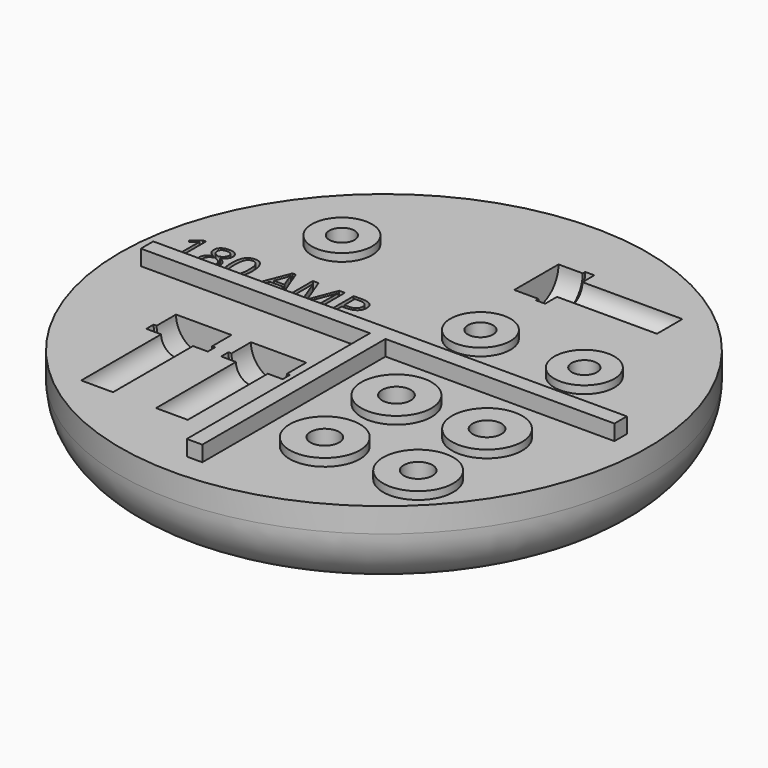
from build123d import *

# Parameters (mm, degrees)
F0_W         = 43
F0_H         = 2
F2_R         = 43.5
F3_DEPTH     = 2
F4_W         = 4
F4_H         = 3.0127849464
F4_H_2       = 58.9872150536
F5_DEPTH     = 4
F6_TEXT_SIZE = 11.6792921391
F7_DEPTH     = 2
F9_R         = 7.75
F10_DEPTH    = 2
F8_R         = 7.75
F11_DEPTH    = 2
F12_R        = 3.25
F13_DEPTH    = 19
F14_R        = 7.75
F15_DEPTH    = 2
F16_R        = 3.25
F17_DEPTH    = 19
F18_R        = 7.75
F19_DEPTH    = 2
F20_R        = 3.25
F21_DEPTH    = 19
F28_R        = 9.05
F32_DEPTH    = 2
F29_R        = 9.05
F30_R        = 9.05
F33_DEPTH    = 2
F31_R        = 9.05
F34_DEPTH    = 2
F35_R        = 3.7
F38_R        = 3.7
F37_R        = 3.7
F36_R        = 3.7
F39_DEPTH    = 19


# Not quite as in the source:
# - Text() gives the source's letters only with a copy of the font that has no kerning and outlines rounded to 1/6400 em; it was checked with that copy


with BuildPart() as f1:
    # F0 (on Front) → F1 (revolve)
    with BuildSketch(Plane.XZ):
        with BuildLine():
            Line((0, -19.3), (0, 0))
            Line((0, 0), (-68, 0))
            Line((-68, 0), (-68, -6.3))
            ThreePointArc((-68, -6.3), (-63.6066017178, -16.9066017178), (-53, -21.3))
            Line((-53, -21.3), (-43, -21.3))
            Line((-43, -21.3), (-43, -19.3))
            Line((-43, -19.3), (0, -19.3))
        make_face()
        with Locations((-21.5, -20.3)):
            Rectangle(F0_W, F0_H)
    revolve(axis=Axis((0, 0, -20.3), (0, 0, 1)))

    # F2 (on face) → F3 (cut)
    with BuildSketch(Plane(origin=(0, 0, -21.3), x_dir=(1, 0, 0), z_dir=(0, 0, -1))):
        Circle(F2_R)
    extrude(amount=-F3_DEPTH, mode=Mode.SUBTRACT)

    # F4 (on face) → F5 (join)
    with BuildSketch(Plane.XY):
        Polygon((-2, -2), (-2, 1.0127849464), (2, 1.0127849464), (2, -2), (60.9872150536, -2), (60.9872150536, 2), (-61.02, 2), (-61.02, -2), align=None)
        with Locations((0, -0.4936075268)):
            Rectangle(F4_W, F4_H)
        with Locations((0, -31.4936075268)):
            Rectangle(F4_W, F4_H_2)
    extrude(amount=F5_DEPTH)

    # F6 (on face) → F7 (cut)
    with BuildSketch(Plane.XY):
        with Locations((-61.5909136832, 6.2500005588)):
            Text('180 AMP', F6_TEXT_SIZE, font='Open Sans', text_align=(TextAlign.LEFT, TextAlign.BOTTOM))
    extrude(amount=-F7_DEPTH, mode=Mode.SUBTRACT)

    # F9 (on face) → F10 (join)
    with BuildSketch(Plane.XY):
        with Locations((-35.4545451701, 30.7954549789)):
            Circle(F9_R)
    extrude(amount=F10_DEPTH)

    # F8 (on face) → F11 (join)
    with BuildSketch(Plane.XY):
        with Locations((-35.4545451701, 30.7954549789)):
            Circle(F8_R)
    extrude(amount=F11_DEPTH)

    # F12 (on face) → F13 (cut)
    with BuildSketch(Plane.XY.offset(2)):
        with Locations((-35.4545451701, 30.7954549789)):
            Circle(F12_R)
    extrude(amount=-F13_DEPTH, mode=Mode.SUBTRACT)

    # F14 (on face) → F15 (join)
    with BuildSketch(Plane.XY):
        with Locations((12.0454542339, 16.0227268934)):
            Circle(F14_R)
    extrude(amount=F15_DEPTH)

    # F16 (on face) → F17 (cut)
    with BuildSketch(Plane.XY.offset(2)):
        with Locations((12.0454542339, 16.0227268934)):
            Circle(F16_R)
    extrude(amount=-F17_DEPTH, mode=Mode.SUBTRACT)

    # F18 (on face) → F19 (join)
    with BuildSketch(Plane.XY):
        with Locations((38.636367768, 16.2500012666)):
            Circle(F18_R)
    extrude(amount=F19_DEPTH)

    # F20 (on face) → F21 (cut)
    with BuildSketch(Plane.XY.offset(2)):
        with Locations((38.636367768, 16.2500012666)):
            Circle(F20_R)
    extrude(amount=-F21_DEPTH, mode=Mode.SUBTRACT)

    # F22 (on face) → F23 (revolve, cut)
    with BuildSketch(Plane.XY):
        Polygon((10.3409079835, 43.9772754908), (4.0909079835, 43.9772754908), (4.0909079835, 36.8522754908), (10.3409079835, 36.8522754908), (10.3409079835, 36.0522754908), (12.6909079835, 36.0522754908), (12.6909079835, 39.8772754908), (38.4409079835, 39.8772754908), (38.4409079835, 43.9772754908), (12.6909079835, 43.9772754908), align=None)
    revolve(axis=Axis((25.5659079835, 43.9772754908, 0), (1, 0, 0)), mode=Mode.SUBTRACT)

    # F24 (on face) → F25 (revolve, cut)
    with BuildSketch(Plane.XY):
        Polygon((-15.925, -22.6136371493), (-15.925, -48.3636371493), (-11.825, -48.3636371493), (-11.825, -22.6136371493), (-8, -22.6136371493), (-8, -20.2636371493), (-8.8, -20.2636371493), (-8.8, -14.0136371493), (-15.925, -14.0136371493), (-15.925, -20.2636371493), align=None)
    revolve(axis=Axis((-15.925, -35.4886371493, 0), (0, -1, 0)), mode=Mode.SUBTRACT)

    # F26 (on face) → F27 (revolve, cut)
    with BuildSketch(Plane.XY):
        Polygon((-28.05, -14.0136371493), (-35.2, -14.0136371493), (-35.2, -20.2636371493), (-35.2, -22.6136371493), (-35.2, -48.3636371493), (-31.1, -48.3636371493), (-31.1, -22.6136371493), (-27.275, -22.6136371493), (-27.275, -20.2636371493), (-28.05, -20.2636371493), align=None)
    revolve(axis=Axis((-35.2, -35.4886371493, 0), (0, -1, 0)), mode=Mode.SUBTRACT)

    # F28 (on face) → F32 (join)
    with BuildSketch(Plane.XY):
        with Locations((16.6225461161, -16.7441392301)):
            Circle(F28_R)
    extrude(amount=F32_DEPTH)

    # F29 (on face) + F30 (on face) → F33 (join)
    with BuildSketch(Plane.XY):
        with Locations((40.0214559379, -16.8149948486)):
            Circle(F29_R)
    with BuildSketch(Plane.XY):
        with Locations((16.8163470961, -40.0522500635)):
            Circle(F30_R)
    extrude(amount=F33_DEPTH)

    # F31 (on face) → F34 (join)
    with BuildSketch(Plane.XY):
        with Locations((40.5137918128, -39.6079486627)):
            Circle(F31_R)
    extrude(amount=F34_DEPTH)

    # F35 (on face) + F38 (on face) + F37 (on face) + F36 (on face) → F39 (cut)
    with BuildSketch(Plane.XY.offset(2)):
        with Locations((16.6225461161, -16.7441392301)):
            Circle(F35_R)
    with BuildSketch(Plane.XY.offset(2)):
        with Locations((40.0214559379, -16.8149948486)):
            Circle(F38_R)
    with BuildSketch(Plane.XY.offset(2)):
        with Locations((40.5137918128, -39.6079486627)):
            Circle(F37_R)
    with BuildSketch(Plane.XY.offset(2)):
        with Locations((16.8163470961, -40.0522500635)):
            Circle(F36_R)
    extrude(amount=-F39_DEPTH, mode=Mode.SUBTRACT)


solid = f1.part
